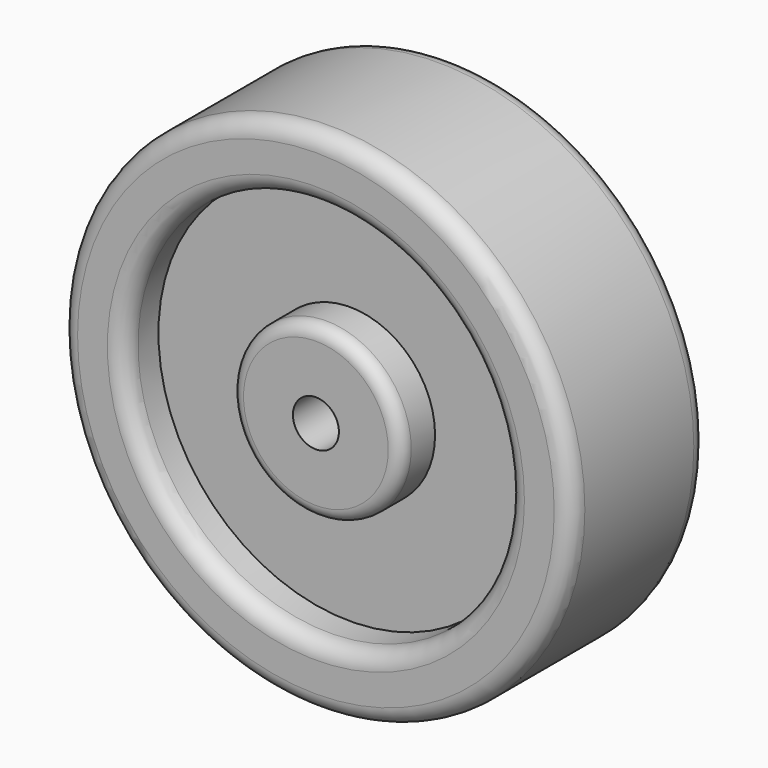
from build123d import *

# Parameters (mm, degrees)
F0_R     = 38.1
F0_R_2   = 3.429
F1_DEPTH = 25.4
F2_R     = 28.575
F2_R_2   = 12.7
F3_DEPTH = 6.35
F4_R     = 28.575
F4_R_2   = 12.7
F5_DEPTH = 6.35
F6_R     = 2.54
F7_R     = 1.905


with BuildPart() as f1:
    # F0 (on Front) → F1 (new body)
    with BuildSketch(Plane.XZ):
        Circle(F0_R)
        Circle(F0_R_2, mode=Mode.SUBTRACT)
    extrude(amount=F1_DEPTH)

    # F2 (on face) → F3 (cut)
    with BuildSketch(Plane.XZ.offset(25.4)):
        Circle(F2_R)
        Circle(F2_R_2, mode=Mode.SUBTRACT)
    extrude(amount=-F3_DEPTH, mode=Mode.SUBTRACT)

    # F4 (on face) → F5 (cut)
    with BuildSketch(Plane(origin=(0, 0, 0), x_dir=(-1, 0, 0), z_dir=(0, 1, 0))):
        Circle(F4_R)
        Circle(F4_R_2, mode=Mode.SUBTRACT)
    extrude(amount=-F5_DEPTH, mode=Mode.SUBTRACT)

    # F6
    f6_edges = [f1.edges().sort_by_distance(p)[0] for p in [
        (28.575, 0, 0),
        (-38.1, 0, 0),
        (-38.1, -25.4, 0),
        (-28.575, -25.4, 0),
    ]]
    fillet(f6_edges, radius=F6_R)

    # F7
    f7_edges = [f1.edges().sort_by_distance(p)[0] for p in [
        (-12.7, -25.4, 0),
        (12.7, 0, 0),
    ]]
    fillet(f7_edges, radius=F7_R)


solid = f1.part
